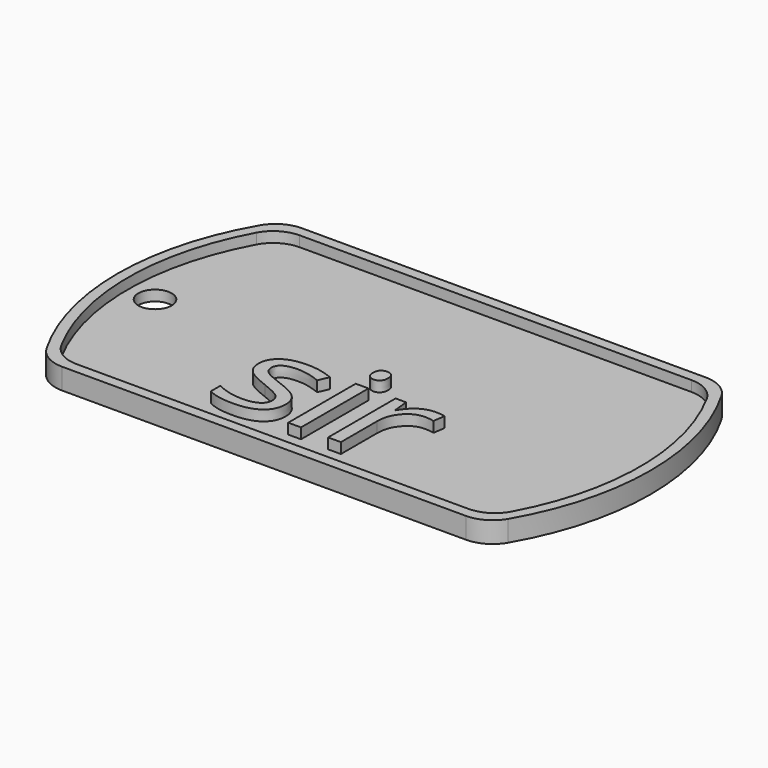
from build123d import *

# Parameters (mm, degrees)
F1_DEPTH     = 1
F3_DEPTH     = 1
F4_R         = 1.5875
F5_DEPTH     = 1
F6_TEXT_SIZE = 15.0260763737
F7_DEPTH     = 1


# Not quite as in the source:
# - Text() gives the source's letters only with a copy of the font that has no kerning and outlines rounded to 1/6400 em; it was checked with that copy


with BuildPart() as f1:
    # F0 (on Top) → F1 (new body)
    with BuildSketch(Plane.XY):
        with BuildLine():
            ThreePointArc((-19.2474145991, 14.2875), (-20.8349145991, 13.862130657), (-21.9970452561, 12.7))
            ThreePointArc((-21.9970452561, 12.7), (-25.4, 0), (-21.9970452561, -12.7))
            ThreePointArc((-21.9970452561, -12.7), (-20.8349145991, -13.862130657), (-19.2474145991, -14.2875))
            Line((-19.2474145991, -14.2875), (19.2474145991, -14.2875))
            ThreePointArc((19.2474145991, -14.2875), (20.8349145991, -13.862130657), (21.9970452561, -12.7))
            ThreePointArc((21.9970452561, -12.7), (25.4, 0), (21.9970452561, 12.7))
            ThreePointArc((21.9970452561, 12.7), (20.8349145991, 13.862130657), (19.2474145991, 14.2875))
            Line((19.2474145991, 14.2875), (-19.2474145991, 14.2875))
        make_face()
    extrude(amount=F1_DEPTH)

    # F2 (on face) → F3 (join)
    with BuildSketch(Plane.XY.offset(1)):
        with BuildLine():
            Line((19.2474145991, 14.2875), (-19.2474145991, 14.2875))
            ThreePointArc((-19.2474145991, 14.2875), (-20.8349145991, 13.862130657), (-21.9970452561, 12.7))
            ThreePointArc((-21.9970452561, 12.7), (-25.4, 0), (-21.9970452561, -12.7))
            ThreePointArc((-21.9970452561, -12.7), (-20.8349145991, -13.862130657), (-19.2474145991, -14.2875))
            Line((-19.2474145991, -14.2875), (19.2474145991, -14.2875))
            ThreePointArc((19.2474145991, -14.2875), (20.8349145991, -13.862130657), (21.9970452561, -12.7))
            ThreePointArc((21.9970452561, -12.7), (25.4, 0), (21.9970452561, 12.7))
            ThreePointArc((21.9970452561, 12.7), (20.8349145991, 13.862130657), (19.2474145991, 14.2875))
        make_face()
        with BuildLine():
            ThreePointArc((-21.4526124879, 11.6252061249), (-20.2856017842, 12.8404540819), (-18.6611352482, 13.2875))
            Line((-18.6611352482, 13.2875), (18.6611352482, 13.2875))
            ThreePointArc((18.6611352482, 13.2875), (20.2856017842, 12.8404540819), (21.4526124879, 11.6252061249))
            ThreePointArc((21.4526124879, 11.6252061249), (24.4, 0), (21.4526124879, -11.6252061249))
            ThreePointArc((21.4526124879, -11.6252061249), (20.2856017842, -12.8404540819), (18.6611352482, -13.2875))
            Line((18.6611352482, -13.2875), (-18.6611352482, -13.2875))
            ThreePointArc((-18.6611352482, -13.2875), (-20.2856017842, -12.8404540819), (-21.4526124879, -11.6252061249))
            ThreePointArc((-21.4526124879, -11.6252061249), (-24.4, 0), (-21.4526124879, 11.6252061249))
        make_face(mode=Mode.SUBTRACT)
    extrude(amount=F3_DEPTH)

    # F4 (on face) → F5 (cut)
    with BuildSketch(Plane.XY.offset(1)):
        with Locations((-21.821282804, 0)):
            Circle(F4_R)
    extrude(amount=-F5_DEPTH, mode=Mode.SUBTRACT)

    # F6 (on face) → F7 (join)
    with BuildSketch(Plane.XY.offset(1)):
        with Locations((-8.9322980569, -10.8187749891)):
            Text('sir', F6_TEXT_SIZE, font='Open Sans', text_align=(TextAlign.LEFT, TextAlign.BOTTOM))
    extrude(amount=F7_DEPTH)


solid = f1.part
